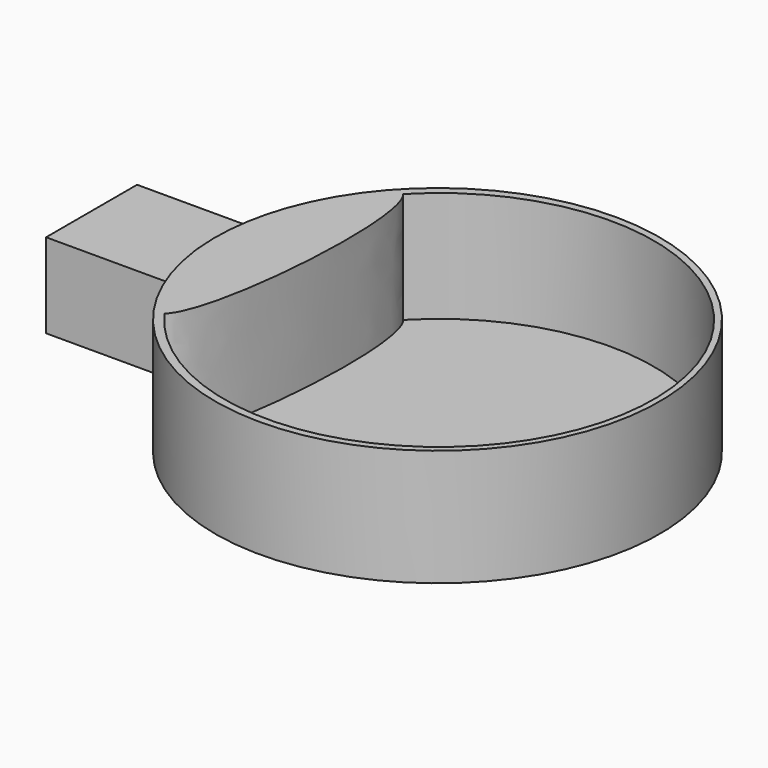
from build123d import *

# Parameters (mm, degrees)
F0_W     = 49
F0_H     = 39
F1_DEPTH = 29
F3_R     = 76.2
F4_DEPTH = 40
F5_R     = 73.66
F6_DEPTH = 38
F2_W     = 35
F2_H     = 25
F7_DEPTH = 147.5
F9_DEPTH = 38


with BuildPart() as f1:
    # F0 (on Top) → F1 (new body)
    with BuildSketch(Plane.XY):
        with Locations((-50.2903954238, 2.6249693376)):
            Rectangle(F0_W, F0_H)
    extrude(amount=F1_DEPTH)

    # F3 (on Top) → F4 (join)
    with BuildSketch(Plane.XY):
        with Locations((50.0179536991, -5.090871723)):
            Circle(F3_R)
    extrude(amount=F4_DEPTH)

    # F5 (on face) → F6 (cut)
    with BuildSketch(Plane.XY.offset(40)):
        with Locations((50.5579536991, -5.090871723)):
            Circle(F5_R)
    extrude(amount=-F6_DEPTH, mode=Mode.SUBTRACT)

    # F2 (on face) → F7 (cut)
    with BuildSketch(Plane(origin=(-74.7903954238, 0, 0), x_dir=(0, -1, 0), z_dir=(-1, 0, 0))):
        with Locations((-2.6249693376, 14.5)):
            Rectangle(F2_W, F2_H)
    extrude(amount=-F7_DEPTH, mode=Mode.SUBTRACT)

    # F8 (on face) → F9 (join)
    with BuildSketch(Plane.XY.offset(2)):
        with BuildLine():
            ThreePointArc((-22.4493461678, -14.8750306624), (-17.8813273172, -32.3279863642), (-9.2079011268, -48.147093073))
            add(Edge.make_bspline(
                [(-2.5791042219, 45.9213687248), (6.562867427, 35.1885122385), (1.3712482781, -38.7284297831), (-9.2079011268, -48.147093073)],
                knots=[0.5957171177, 0.5957171177, 0.5957171177, 0.5957171177, 1, 1, 1, 1], degree=3))
            ThreePointArc((-2.5791042219, 45.9213687248), (-11.9603198587, 33.8611637996), (-18.6515612509, 20.1249693376))
            Line((-18.6515612509, 20.1249693376), (-21.8889399872, 20.1249693376))
            ThreePointArc((-21.8889399872, 20.1249693376), (-22.927932873, 16.9395080336), (-23.8258859148, 13.7114513007))
            add(Edge.make_bspline(
                [(-25.7903954238, -12.9307361878), (-26.0689147995, -8.6981558447), (-26.1124652464, 0.3286887969), (-24.7810032726, 9.273748372), (-23.8258859148, 13.7114513007)],
                knots=[0.2496191663, 0.2496191663, 0.2496191663, 0.2496191663, 0.2970853564, 0.3479233847, 0.3479233847, 0.3479233847, 0.3479233847], degree=3))
            Line((-25.7903954238, -12.9307361878), (-25.7903954238, -12.8067127836))
            ThreePointArc((-25.7903954238, -12.8067127836), (-25.6779062067, -13.8416884355), (-25.5512876221, -14.8750306624))
            Line((-25.5512876221, -14.8750306624), (-22.4493461678, -14.8750306624))
        make_face()
    extrude(amount=F9_DEPTH)


solid = f1.part
